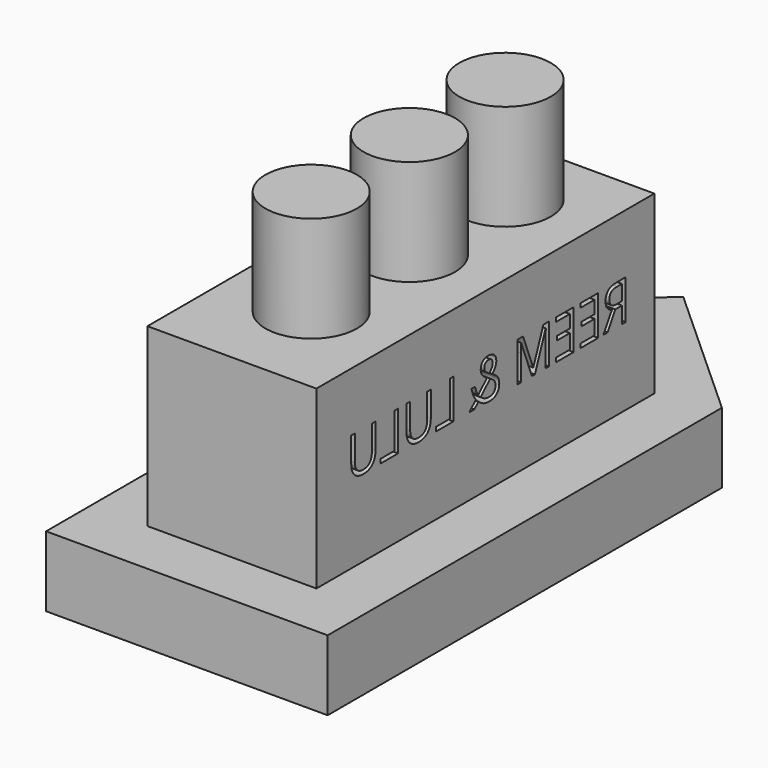
from build123d import *

# Parameters (mm, degrees)
F1_DEPTH     = 10
F2_W         = 24
F2_H         = 60
F3_DEPTH     = 25
F4_R         = 6.5
F5_DEPTH     = 15
F6_TEXT_SIZE = 7.8728534173
F7_DEPTH     = 25


# Not quite as in the source:
# - Text() gives the source's letters only with a copy of the font that has no kerning and outlines rounded to 1/6400 em; it was checked with that copy


with BuildPart() as f1:
    # F0 (on Top) → F1 (new body)
    with BuildSketch(Plane.XY):
        Polygon((0, 66.0628745109), (-20, 47.9245173637), (-20, -22.0754826363), (20, -22.0754826363), (20, 47.9245173637), align=None)
    extrude(amount=F1_DEPTH)

    # F2 (on face) → F3 (join)
    with BuildSketch(Plane.XY.offset(10)):
        with Locations((0, 15.9245173637)):
            Rectangle(F2_W, F2_H)
    extrude(amount=F3_DEPTH)

    # F4 (on face) → F5 (join)
    with BuildSketch(Plane.XY.offset(35)):
        with Locations((0, 34.4245173637)):
            Circle(F4_R)
        with Locations((0, 17.4245173637)):
            Circle(F4_R)
        Circle(F4_R)
    extrude(amount=F5_DEPTH)

    # F6 (on face) → F7 (cut)
    with BuildSketch(Plane(origin=(-12, 0, 0), x_dir=(0, -1, 0), z_dir=(-1, 0, 0))):
        with Locations((-41.5988539308, 20.9965360464)):
            Text('REEM & LULU', F6_TEXT_SIZE, font='Open Sans', text_align=(TextAlign.LEFT, TextAlign.BOTTOM))
    extrude(amount=-F7_DEPTH, mode=Mode.SUBTRACT)


solid = f1.part
